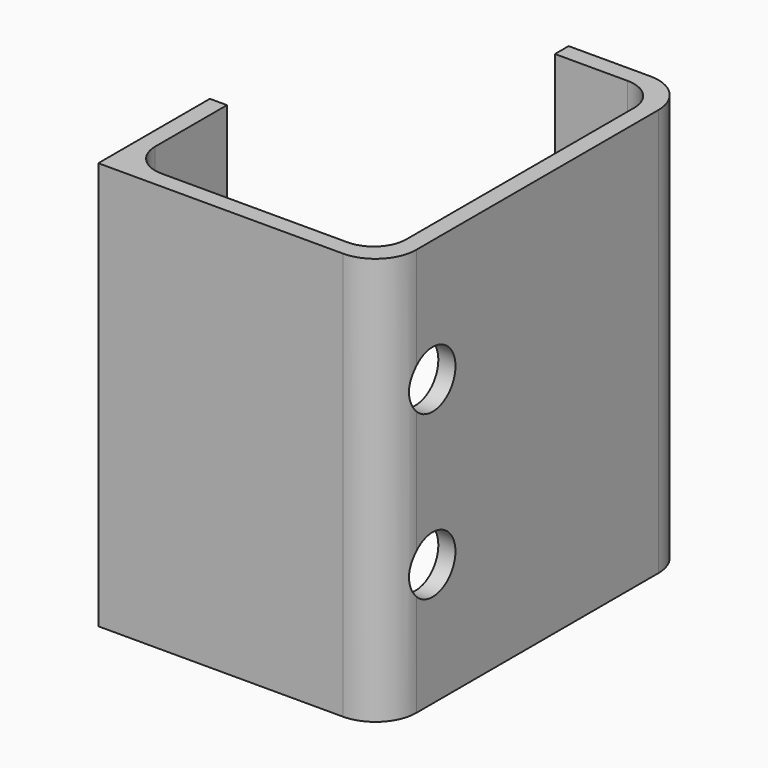
from build123d import *

# Parameters (mm, degrees)
F1_DEPTH      = 50
F2_R          = 1.25
F3_DEPTH      = 32.901
F2_R_2        = 3.5
F4_DEPTH      = 2.1
F4_DEPTH_BACK = 10
F5_T1_DEPTH   = 75


# Not quite as in the source:
# - a fillet or chamfer that OpenCascade refuses, or shapes differently, is made with other operations: its cross-section is extruded or revolved along the edge and cut away or added


with BuildPart() as f1:
    # F0 (on Top) → F1 (new body)
    with BuildSketch(Plane.XY):
        with BuildLine():
            ThreePointArc((0, 4), (-1.1715728753, 1.1715728753), (-4, 0))
            Line((-4, 0), (-26.8, 0))
            ThreePointArc((-26.8, 0), (-29.6284271247, 1.1715728753), (-30.8, 4))
            Line((-30.8, 4), (-30.8, 15))
            Line((-30.8, 15), (-32.9, 15))
            Line((-32.9, 15), (-32.9, -2.1))
            Line((-32.9, -2.1), (2.1, -2.1))
            Line((2.1, -2.1), (2.1, 45))
            Line((2.1, 45), (-12.9, 45))
            Line((-12.9, 45), (-12.9, 42.9))
            Line((-12.9, 42.9), (-4, 42.9))
            ThreePointArc((-4, 42.9), (-1.1715728753, 41.7284271247), (0, 38.9))
            Line((0, 38.9), (0, 4))
        make_face()
    extrude(amount=F1_DEPTH)

    # F2 (on Right) → F3 (cut, through all)
    with BuildSketch(Plane.YZ):
        with Locations((5.4, 35)):
            Circle(F2_R)
        with Locations((5.4, 15)):
            Circle(F2_R)
    extrude(amount=-F3_DEPTH, mode=Mode.SUBTRACT)

    # F2 (on Right) → F4 (cut, two sides)
    with BuildSketch(Plane.YZ) as f4_sk:
        with Locations((5.4, 35)):
            Circle(F2_R_2)
        with Locations((5.4, 35)):
            Circle(F2_R, mode=Mode.SUBTRACT)
        with Locations((5.4, 15)):
            Circle(F2_R_2)
        with Locations((5.4, 15)):
            Circle(F2_R, mode=Mode.SUBTRACT)
        with Locations((5.4, 15)):
            Circle(F2_R)
        with Locations((5.4, 35)):
            Circle(F2_R)
    extrude(amount=F4_DEPTH, mode=Mode.SUBTRACT)
    extrude(f4_sk.sketch, amount=-F4_DEPTH_BACK, mode=Mode.SUBTRACT)

    # F5: fillet of radius 5 on 2 edges, made by hand

    # F5_s2 → F5_t1 (cut)
    with BuildSketch(Plane.XY.offset(-12.5)):
        with BuildLine():
            ThreePointArc((2.1, 40), (0.6355339059, 43.5355339059), (-2.9, 45))
            Line((-2.9, 45), (2.1, 45))
            Line((2.1, 45), (2.1, 40))
        make_face()
        with BuildLine():
            ThreePointArc((-2.9, -2.1), (0.6355339059, -0.6355339059), (2.1, 2.9))
            Line((2.1, 2.9), (2.1, -2.1))
            Line((2.1, -2.1), (-2.9, -2.1))
        make_face()
    extrude(amount=F5_T1_DEPTH, mode=Mode.SUBTRACT)


solid = f1.part
